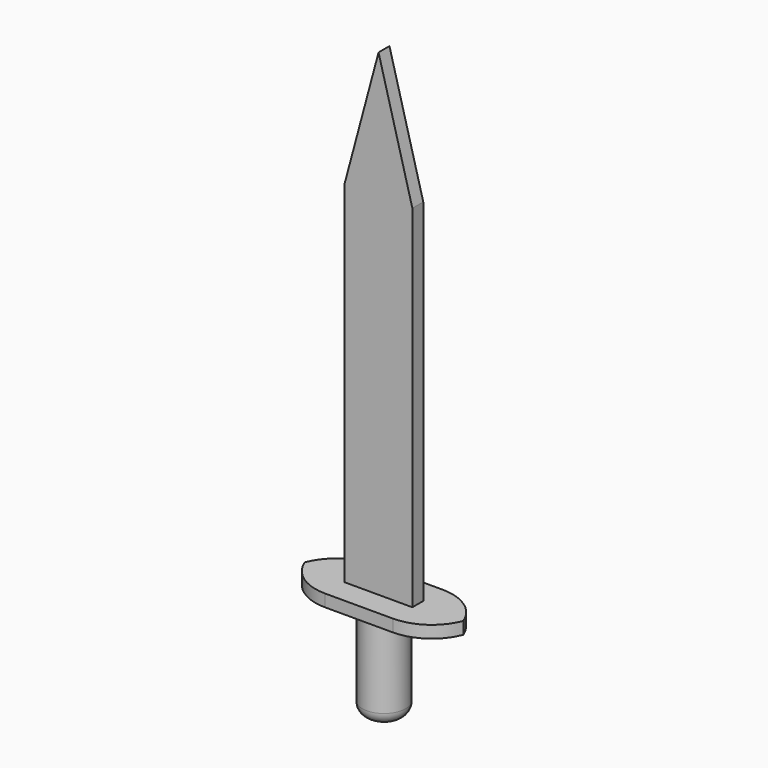
from build123d import *

# Parameters (mm, degrees)
F0_R        = 2.25
F1_DEPTH    = 10
F2_W        = 17.2
F2_H        = 6.5
F2_R        = 2.25
F3_DEPTH    = 1.27
F4_W        = 7.04
F4_H        = 1.42
F5_DEPTH    = 50.8
F6_T1_DEPTH = 75.2661578682
F7_T1_DEPTH = 26.67
F8_R        = 1.27


# Not quite as in the source:
# - a fillet or chamfer that OpenCascade refuses, or shapes differently, is made with other operations: its cross-section is extruded or revolved along the edge and cut away or added


with BuildPart() as f1:
    # F0 (on Top) → F1 (new body)
    with BuildSketch(Plane.XY):
        Circle(F0_R)
    extrude(amount=F1_DEPTH)

    # F2 (on face) → F3 (join)
    with BuildSketch(Plane.XY.offset(10)):
        Rectangle(F2_W, F2_H)
        Circle(F2_R, mode=Mode.SUBTRACT)
        Circle(F2_R)
    extrude(amount=F3_DEPTH)

    # F4 (on face) → F5 (join)
    with BuildSketch(Plane.XY.offset(11.27)):
        Rectangle(F4_W, F4_H)
    extrude(amount=F5_DEPTH)

    # F6: chamfer of 3.81 x 14.2191135768 on 2 edges, made by hand

    # F6_s2 → F6_t1 (cut)
    with BuildSketch(Plane.XZ.offset(-37.6330789341)):
        Polygon((-3.52, 47.8508864232), (0.29, 62.07), (-3.52, 62.07), align=None)
        Polygon((3.52, 47.8508864232), (-0.29, 62.07), (3.52, 62.07), align=None)
    extrude(amount=F6_T1_DEPTH, mode=Mode.SUBTRACT)

    # F7: fillet of radius 5.08 on 4 edges, made by hand

    # F7_s2 → F7_t1 (cut)
    with BuildSketch(Plane.XY.offset(-2.7)):
        with BuildLine():
            ThreePointArc((-8.6, 1.83), (-7.1121024484, -1.7621024484), (-3.52, -3.25))
            Line((-3.52, -3.25), (-8.6, -3.25))
            Line((-8.6, -3.25), (-8.6, 1.83))
        make_face()
        with BuildLine():
            ThreePointArc((-3.52, 3.25), (-7.1121024484, 1.7621024484), (-8.6, -1.83))
            Line((-8.6, -1.83), (-8.6, 3.25))
            Line((-8.6, 3.25), (-3.52, 3.25))
        make_face()
        with BuildLine():
            ThreePointArc((8.6, 1.83), (7.1121024484, -1.7621024484), (3.52, -3.25))
            Line((3.52, -3.25), (8.6, -3.25))
            Line((8.6, -3.25), (8.6, 1.83))
        make_face()
        with BuildLine():
            ThreePointArc((3.52, 3.25), (7.1121024484, 1.7621024484), (8.6, -1.83))
            Line((8.6, -1.83), (8.6, 3.25))
            Line((8.6, 3.25), (3.52, 3.25))
        make_face()
    extrude(amount=F7_T1_DEPTH, mode=Mode.SUBTRACT)

    # F8
    f8_edges = [f1.edges().sort_by_distance(p)[0] for p in [
        (-2.25, 0, 0),
    ]]
    fillet(f8_edges, radius=F8_R)


solid = f1.part
